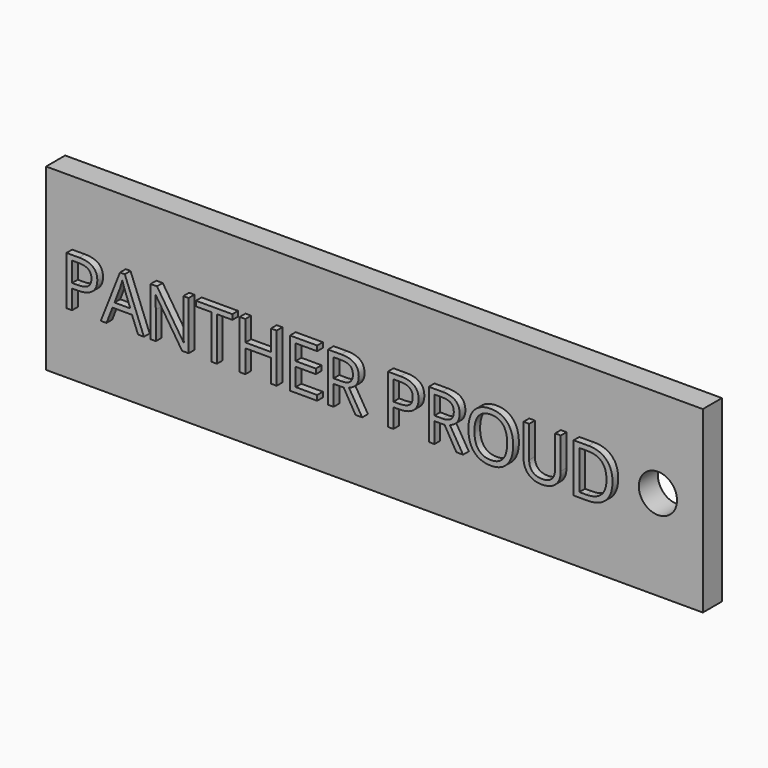
from build123d import *

# Parameters (mm, degrees)
F0_W         = 69.85
F0_H         = 19.05
F0_R         = 2.032
F1_DEPTH     = 2.54
F2_TEXT_SIZE = 7.2498566523
F3_DEPTH     = 0.762


# Not quite as in the source:
# - Text() gives the source's letters only with a copy of the font that has no kerning and outlines rounded to 1/6400 em; it was checked with that copy


with BuildPart() as f1:
    # F0 (on Front) → F1 (new body)
    with BuildSketch(Plane.XZ):
        with Locations((-21.7030521452, 5.3550637081)):
            Rectangle(F0_W, F0_H)
        with Locations((8.4467478548, 5.4386528209)):
            Circle(F0_R, mode=Mode.SUBTRACT)
    extrude(amount=F1_DEPTH)

    # F2 (on face) → F3 (join)
    with BuildSketch(Plane.XZ.offset(2.54)):
        with Locations((-54.5650445856, 2.8269572649)):
            Text('PANTHER PROUD', F2_TEXT_SIZE, font='Open Sans', text_align=(TextAlign.LEFT, TextAlign.BOTTOM))
    extrude(amount=F3_DEPTH)


solid = f1.part
